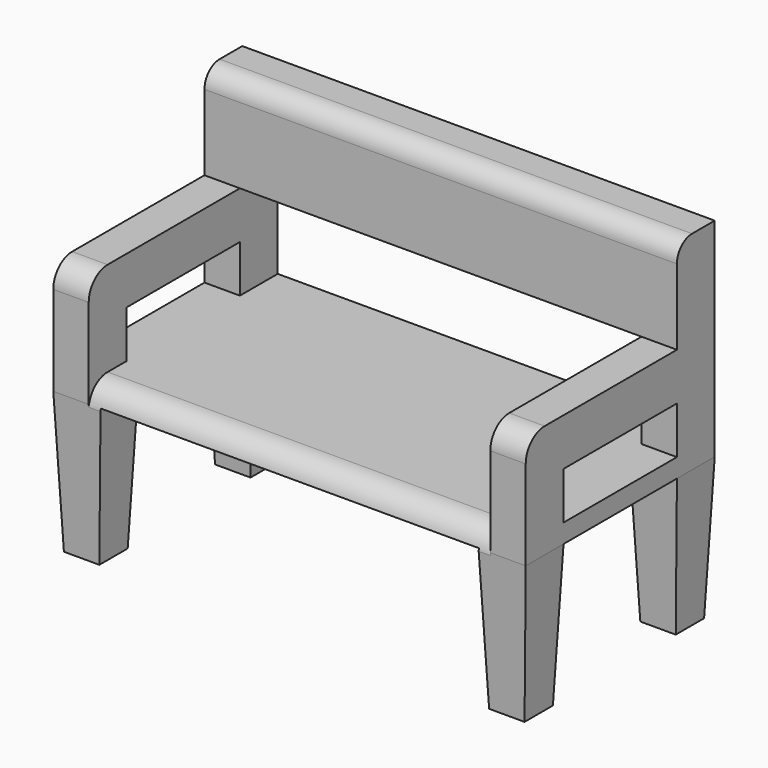
from build123d import *

# Parameters (mm, degrees)
F0_W         = 200
F0_H         = 100
F1_DEPTH     = 8
F2_W         = 20
F2_H         = 20
F4_W         = 15
F4_H         = 15
F8_W         = 15
F8_H         = 20
F9_DEPTH     = 80
F11_W        = 20
F11_H        = 40
F12_DEPTH    = 170
F14_DEPTH    = 80
F15_W        = 15
F15_H        = 20
F16_DEPTH    = 20
F18_R        = 10
F19_R        = 10
F20_T1_DEPTH = 170
F21_R        = 8


# Not quite as in the source:
# - a fillet or chamfer that OpenCascade refuses, or shapes differently, is made with other operations: its cross-section is extruded or revolved along the edge and cut away or added


with BuildPart() as f1:
    # F0 (on Top) → F1 (new body)
    with BuildSketch(Plane.XY):
        Rectangle(F0_W, F0_H)
    extrude(amount=F1_DEPTH)

    # F2 (on face) → F5 section 0
    with BuildSketch(Plane(origin=(0, 0, 0), x_dir=(1, 0, 0), z_dir=(0, 0, -1))):
        with Locations((-90, 40)):
            Rectangle(F2_W, F2_H)
    # F4 (on offset) → F5 section 1
    with BuildSketch(Plane.XY.offset(-60)):
        with Locations((-90, -40)):
            Rectangle(F4_W, F4_H)
    loft()

    # F6: F1 across plane


with BuildPart() as f1_1:
    add(f1.part)
    add(f1.part.mirror(Plane.XZ))

    # F7: F1 across plane


with BuildPart() as f1_2:
    add(f1_1.part)
    add(f1_1.part.mirror(Plane.YZ))

    # F8 (on face) → F9 (join)
    with BuildSketch(Plane.XY.offset(8)):
        with Locations((-92.5, 40)):
            Rectangle(F8_W, F8_H)
    extrude(amount=F9_DEPTH)

    # F10: F1 across plane


with BuildPart() as f1_3:
    add(f1_2.part)
    add(f1_2.part.mirror(Plane.YZ))

    # F11 (on face) → F12 (join)
    with BuildSketch(Plane.YZ.offset(-85)):
        with Locations((40, 68)):
            Rectangle(F11_W, F11_H)
    extrude(amount=F12_DEPTH)

    # F13 (on face) → F14 (join)
    with BuildSketch(Plane.XZ.offset(-30)):
        Polygon((-85, 28), (-85, 48), (-92.5, 48), (-100, 48), (-100, 28), align=None)
    extrude(amount=F14_DEPTH)

    # F15 (on face) → F16 (join)
    with BuildSketch(Plane(origin=(0, 0, 28), x_dir=(1, 0, 0), z_dir=(0, 0, -1))):
        with Locations((-92.5, 40)):
            Rectangle(F15_W, F15_H)
    extrude(amount=F16_DEPTH)

    # F17: F1 across plane


with BuildPart() as f1_4:
    add(f1_3.part)
    add(f1_3.part.mirror(Plane.YZ))

    # F18
    f18_edges = [f1_4.edges().sort_by_distance(p)[0] for p in [
        (92.5, -50, 48),
    ]]
    fillet(f18_edges, radius=F18_R)

    # F19
    f19_edges = [f1_4.edges().sort_by_distance(p)[0] for p in [
        (-92.5, -50, 48),
    ]]
    fillet(f19_edges, radius=F19_R)

    # F20: fillet of radius 10 on 1 edges, made by hand

    # F20_s2 → F20_t1 (cut)
    with BuildSketch(Plane.YZ.offset(-85)):
        with BuildLine():
            ThreePointArc((-50, -2), (-47.0710678119, 5.0710678119), (-40, 8))
            Line((-40, 8), (-50, 8))
            Line((-50, 8), (-50, -2))
        make_face()
    extrude(amount=F20_T1_DEPTH, mode=Mode.SUBTRACT)

    # F21
    f21_edges = [f1_4.edges().sort_by_distance(p)[0] for p in [
        (0, 30, 88),
    ]]
    fillet(f21_edges, radius=F21_R)


solid = f1_4.part
